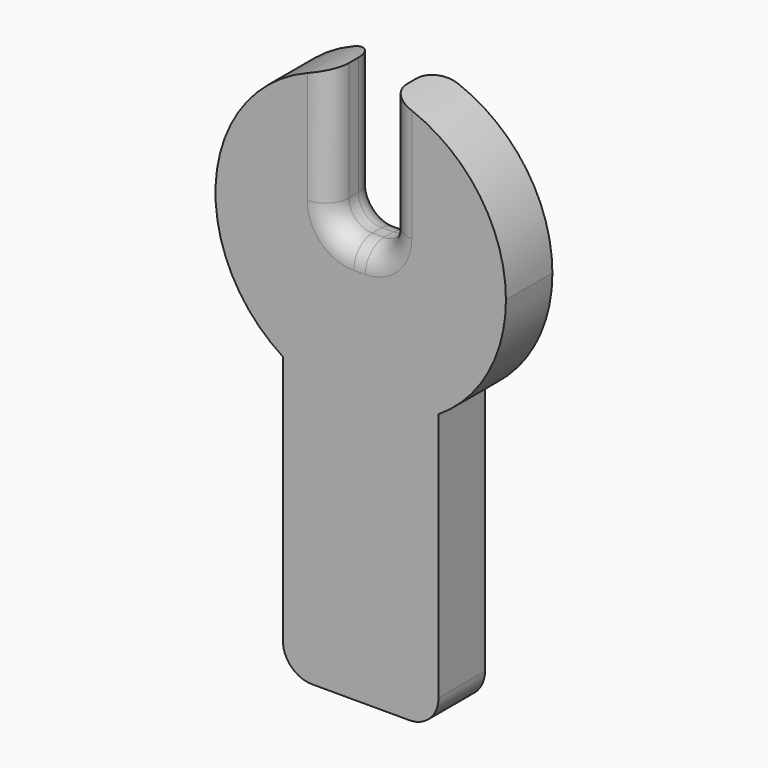
from build123d import *

# Parameters (mm, degrees)
F1_DEPTH = 12.7
F2_R     = 5.08


# Not quite as in the source:
# - a feature names something its author has since deleted; it is built from what else it names


with BuildPart() as f1:
    # F0 (on Front) → F1 (new body)
    with BuildSketch(Plane.XZ):
        with BuildLine():
            ThreePointArc((-6.6039999947, 74.8653914212), (-31.2484265209, 49.4310412723), (-17.0128613258, 17.0026184017))
            Line((-17.0128613258, 17.0026184017), (17.0128613258, 17.0026184017))
            ThreePointArc((17.0128613258, 17.0026184017), (27.8228399619, 28.5143091682), (31.75, 43.8098011987))
            ThreePointArc((31.75, 43.8098011987), (24.5113290151, 63.9904168958), (6.0960000053, 74.9690900855))
            Line((6.0960000053, 74.9690900855), (6.0960000053, 62.4722737233))
            Line((6.0960000053, 62.4722737233), (6.0960000053, 43.7620282173))
            Line((6.0960000053, 43.7620282173), (-6.6039999947, 43.7620282173))
            Line((-6.6039999947, 43.7620282173), (-6.6039999947, 62.4722737233))
            Line((-6.6039999947, 62.4722737233), (-6.6039999947, 74.8653914212))
        make_face()
        with BuildLine():
            ThreePointArc((17.0128613258, 17.0026184017), (0, 12.0598011987), (-17.0128613258, 17.0026184017))
            Line((-17.0128613258, 17.0026184017), (-17.0128613258, -37.617602489))
            ThreePointArc((-17.0128613258, -37.617602489), (-15.1529893863, -42.1077305495), (-10.6628613258, -43.967602489))
            Line((-10.6628613258, -43.967602489), (10.6628613258, -43.967602489))
            ThreePointArc((10.6628613258, -43.967602489), (15.1529893863, -42.1077305495), (17.0128613258, -37.617602489))
            Line((17.0128613258, -37.617602489), (17.0128613258, 17.0026184017))
        make_face()
        with BuildLine():
            Line((17.0128613258, 17.0026184017), (-17.0128613258, 17.0026184017))
            ThreePointArc((-17.0128613258, 17.0026184017), (0, 12.0598011987), (17.0128613258, 17.0026184017))
        make_face()
    extrude(amount=F1_DEPTH)

    # F2
    f2_edges = [f1.edges().sort_by_distance(p)[0] for p in [
        (6.096, -6.35, 43.762028),
        (-6.604, -6.35, 43.762028),
        (-0.254, 0, 43.762028),
        (-0.254, -12.7, 43.762028),
        (6.096, 0, 59.365559),
        (6.096, -12.7, 59.365559),
        (-6.604, 0, 59.31371),
        (-6.604, -12.7, 59.31371),
    ]]
    fillet(f2_edges, radius=F2_R)


solid = f1.part
